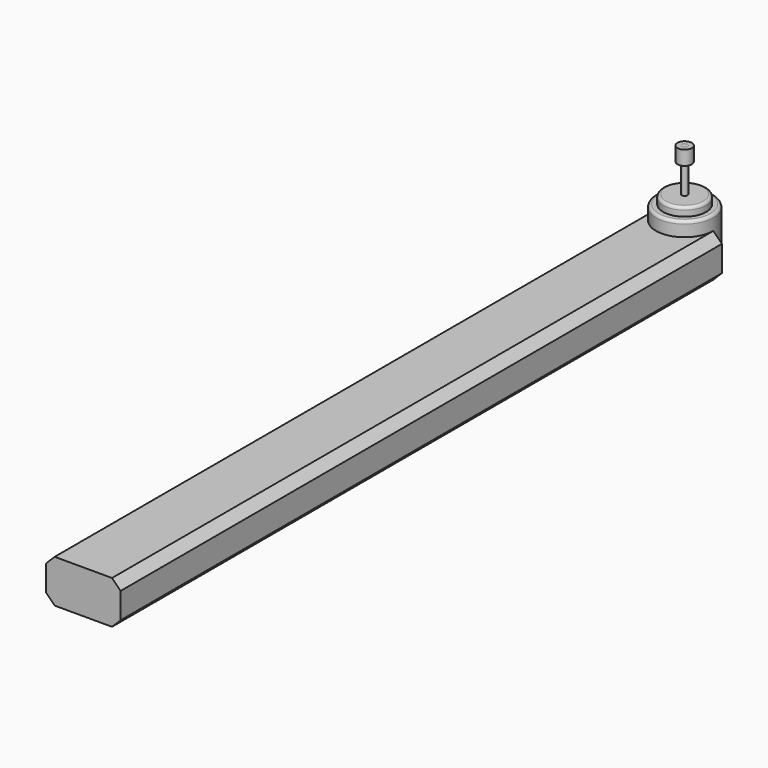
from build123d import *

# Parameters (mm, degrees)
F0_R      = 10
F1_DEPTH  = 20
F2_R      = 7.5
F3_DEPTH  = 3
F4_R      = 1
F5_DEPTH  = 15
F6_R      = 2.5
F6_R_2    = 1
F7_DEPTH  = 5
F8_R      = 1
F10_DEPTH = 15
F9_W      = 26
F9_H      = 250
F11_DEPTH = 15
F12_SIZE  = 3


with BuildPart() as f1:
    # F0 (on Top) → F1 (new body)
    with BuildSketch(Plane.XY):
        with Locations((-51.0874686381, 0)):
            Circle(F0_R)
    extrude(amount=F1_DEPTH)

    # F2 (on face) → F3 (join)
    with BuildSketch(Plane.XY.offset(20)):
        with Locations((-51.0874686381, 0)):
            Circle(F2_R)
    extrude(amount=F3_DEPTH)

    # F4 (on face) → F5 (join)
    with BuildSketch(Plane.XY.offset(23)):
        with Locations((-51.0874686381, 0)):
            Circle(F4_R)
    extrude(amount=F5_DEPTH)

    # F8
    f8_edges = [f1.edges().sort_by_distance(p)[0] for p in [
        (-61.087469, 0, 0),
        (-61.087469, 0, 20),
        (-58.587469, 0, 23),
    ]]
    fillet(f8_edges, radius=F8_R)


with BuildPart() as f7:
    # F6 (on face) → F7 (new body)
    with BuildSketch(Plane.XY.offset(38)):
        with Locations((-51.0874686381, 0)):
            Circle(F6_R)
        with Locations((-51.0874686381, 0)):
            Circle(F6_R_2, mode=Mode.SUBTRACT)
    extrude(amount=-F7_DEPTH)


with BuildPart() as f10:
    # F9 (on Top) → F10 (new body)
    with BuildSketch(Plane.XY):
        with BuildLine():
            Line((-38.0874686381, 0), (-41.0874686381, 0))
            ThreePointArc((-41.0874686381, 0), (-51.0874686381, -10), (-61.0874686381, 0))
            Line((-61.0874686381, 0), (-64.0874686381, 0))
            Line((-64.0874686381, 0), (-64.0874686381, -12.2324628755))
            Line((-64.0874686381, -12.2324628755), (-38.0874686381, -12.2324628755))
            Line((-38.0874686381, -12.2324628755), (-38.0874686381, 0))
        make_face()
    extrude(amount=F10_DEPTH)

    # F9 (on Top) → F11 (join)
    with BuildSketch(Plane.XY):
        with Locations((-51.0874686381, -137.2324628755)):
            Rectangle(F9_W, F9_H)
    extrude(amount=F11_DEPTH)

    # F12
    f12_edges = [f10.edges().sort_by_distance(p)[0] for p in [
        (-64.087469, -131.116231, 15),
        (-38.087469, -131.116231, 15),
        (-38.087469, -131.116231, 0),
        (-64.087469, -131.116231, 0),
    ]]
    chamfer(f12_edges, length=F12_SIZE)


solid = Compound([f1.part, f7.part, f10.part])
